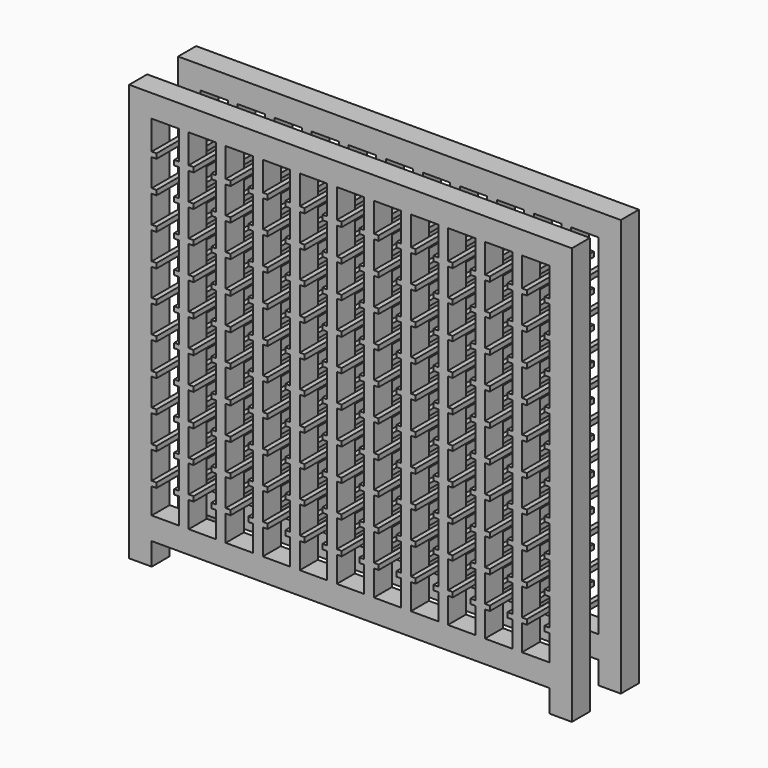
from build123d import *

# Parameters (mm, degrees)
F0_W          = 1568.45
F0_H          = 88.9
F1_DEPTH      = 88.9
F2_W          = 38.1
F2_H          = 1377.95
F3_DEPTH      = 88.9
F6_W          = 19.05
F6_H          = 19.05
F7_DEPTH      = 165.1
F7_DEPTH_BACK = 165.1


with BuildPart() as f1:
    # F0 (on Front) → F1 (new body)
    with BuildSketch(Plane.XZ):
        Polygon((0, 1644.65), (0, 0), (88.9, 0), (88.9, 88.9), (88.9, 177.8), (88.9, 1555.75), (88.9, 1644.65), align=None)
        with Locations((873.125, 133.35)):
            Rectangle(F0_W, F0_H)
        with Locations((873.125, 1600.2)):
            Rectangle(F0_W, F0_H)
        Polygon((1657.35, 177.8), (1657.35, 88.9), (1657.35, 0), (1746.25, 0), (1746.25, 1644.65), (1657.35, 1644.65), (1657.35, 1555.75), align=None)
    extrude(amount=F1_DEPTH)

    # F2 (on face) → F3 (join)
    with BuildSketch(Plane.XZ.offset(88.9)):
        Polygon((1746.25, 1644.65), (0, 1644.65), (0, 0), (88.9, 0), (88.9, 88.9), (1657.35, 88.9), (1657.35, 0), (1746.25, 0), align=None)
        Polygon((88.9, 1555.75), (196.85, 1555.75), (234.95, 1555.75), (342.9, 1555.75), (381, 1555.75), (488.95, 1555.75), (527.05, 1555.75), (635, 1555.75), (673.1, 1555.75), (781.05, 1555.75), (819.15, 1555.75), (927.1, 1555.75), (965.2, 1555.75), (1073.15, 1555.75), (1111.25, 1555.75), (1219.2, 1555.75), (1257.3, 1555.75), (1365.25, 1555.75), (1403.35, 1555.75), (1511.3, 1555.75), (1549.4, 1555.75), (1657.35, 1555.75), (1657.35, 177.8), (1549.4, 177.8), (1511.3, 177.8), (1403.35, 177.8), (1365.25, 177.8), (1257.3, 177.8), (1219.2, 177.8), (1111.25, 177.8), (1073.15, 177.8), (965.2, 177.8), (927.1, 177.8), (819.15, 177.8), (781.05, 177.8), (673.1, 177.8), (635, 177.8), (527.05, 177.8), (488.95, 177.8), (381, 177.8), (342.9, 177.8), (234.95, 177.8), (196.85, 177.8), (88.9, 177.8), align=None, mode=Mode.SUBTRACT)
        with Locations((215.9, 866.775)):
            Rectangle(F2_W, F2_H)
        with Locations((361.95, 866.775)):
            Rectangle(F2_W, F2_H)
        with Locations((508, 866.775)):
            Rectangle(F2_W, F2_H)
        with Locations((654.05, 866.775)):
            Rectangle(F2_W, F2_H)
        with Locations((800.1, 866.775)):
            Rectangle(F2_W, F2_H)
        with Locations((946.15, 866.775)):
            Rectangle(F2_W, F2_H)
        with Locations((1092.2, 866.775)):
            Rectangle(F2_W, F2_H)
        with Locations((1238.25, 866.775)):
            Rectangle(F2_W, F2_H)
        with Locations((1384.3, 866.775)):
            Rectangle(F2_W, F2_H)
        with Locations((1530.35, 866.775)):
            Rectangle(F2_W, F2_H)
    extrude(amount=-F3_DEPTH)


with BuildPart() as f5_1:
    # F5: instance of F1
    add(f1.part.mirror(Plane(origin=(873.125, 76.2, 854.9186148301), x_dir=(1, 0, 0), z_dir=(0, -1, 0))))


with BuildPart() as f1_1:
    add(f1.part)

    add(f5_1.part)  # F7 merges F5_1
    # F6 (on offset) → F7 (join, two sides)
    with BuildSketch(Plane.XZ.offset(-76.2)) as f7_sk:
        with Locations((98.425, 288.925)):
            Rectangle(F6_W, F6_H)
        with Locations((98.425, 415.925)):
            Rectangle(F6_W, F6_H)
        with Locations((98.425, 542.925)):
            Rectangle(F6_W, F6_H)
        with Locations((98.425, 669.925)):
            Rectangle(F6_W, F6_H)
        with Locations((98.425, 796.925)):
            Rectangle(F6_W, F6_H)
        with Locations((98.425, 923.925)):
            Rectangle(F6_W, F6_H)
        with Locations((98.425, 1050.925)):
            Rectangle(F6_W, F6_H)
        with Locations((98.425, 1177.925)):
            Rectangle(F6_W, F6_H)
        with Locations((98.425, 1304.925)):
            Rectangle(F6_W, F6_H)
        with Locations((244.475, 288.925)):
            Rectangle(F6_W, F6_H)
        with Locations((244.475, 415.925)):
            Rectangle(F6_W, F6_H)
        with Locations((244.475, 542.925)):
            Rectangle(F6_W, F6_H)
        with Locations((244.475, 669.925)):
            Rectangle(F6_W, F6_H)
        with Locations((244.475, 796.925)):
            Rectangle(F6_W, F6_H)
        with Locations((244.475, 923.925)):
            Rectangle(F6_W, F6_H)
        with Locations((244.475, 1050.925)):
            Rectangle(F6_W, F6_H)
        with Locations((244.475, 1177.925)):
            Rectangle(F6_W, F6_H)
        with Locations((244.475, 1304.925)):
            Rectangle(F6_W, F6_H)
        with Locations((390.525, 288.925)):
            Rectangle(F6_W, F6_H)
        with Locations((390.525, 415.925)):
            Rectangle(F6_W, F6_H)
        with Locations((390.525, 542.925)):
            Rectangle(F6_W, F6_H)
        with Locations((390.525, 669.925)):
            Rectangle(F6_W, F6_H)
        with Locations((390.525, 796.925)):
            Rectangle(F6_W, F6_H)
        with Locations((390.525, 923.925)):
            Rectangle(F6_W, F6_H)
        with Locations((390.525, 1050.925)):
            Rectangle(F6_W, F6_H)
        with Locations((390.525, 1177.925)):
            Rectangle(F6_W, F6_H)
        with Locations((390.525, 1304.925)):
            Rectangle(F6_W, F6_H)
        with Locations((536.575, 288.925)):
            Rectangle(F6_W, F6_H)
        with Locations((536.575, 415.925)):
            Rectangle(F6_W, F6_H)
        with Locations((536.575, 542.925)):
            Rectangle(F6_W, F6_H)
        with Locations((536.575, 669.925)):
            Rectangle(F6_W, F6_H)
        with Locations((536.575, 796.925)):
            Rectangle(F6_W, F6_H)
        with Locations((536.575, 923.925)):
            Rectangle(F6_W, F6_H)
        with Locations((536.575, 1050.925)):
            Rectangle(F6_W, F6_H)
        with Locations((536.575, 1177.925)):
            Rectangle(F6_W, F6_H)
        with Locations((536.575, 1304.925)):
            Rectangle(F6_W, F6_H)
        with Locations((682.625, 288.925)):
            Rectangle(F6_W, F6_H)
        with Locations((682.625, 415.925)):
            Rectangle(F6_W, F6_H)
        with Locations((682.625, 542.925)):
            Rectangle(F6_W, F6_H)
        with Locations((682.625, 669.925)):
            Rectangle(F6_W, F6_H)
        with Locations((682.625, 796.925)):
            Rectangle(F6_W, F6_H)
        with Locations((682.625, 923.925)):
            Rectangle(F6_W, F6_H)
        with Locations((682.625, 1050.925)):
            Rectangle(F6_W, F6_H)
        with Locations((682.625, 1177.925)):
            Rectangle(F6_W, F6_H)
        with Locations((682.625, 1304.925)):
            Rectangle(F6_W, F6_H)
        with Locations((828.675, 288.925)):
            Rectangle(F6_W, F6_H)
        with Locations((828.675, 415.925)):
            Rectangle(F6_W, F6_H)
        with Locations((828.675, 542.925)):
            Rectangle(F6_W, F6_H)
        with Locations((828.675, 669.925)):
            Rectangle(F6_W, F6_H)
        with Locations((828.675, 796.925)):
            Rectangle(F6_W, F6_H)
        with Locations((828.675, 923.925)):
            Rectangle(F6_W, F6_H)
        with Locations((828.675, 1050.925)):
            Rectangle(F6_W, F6_H)
        with Locations((828.675, 1177.925)):
            Rectangle(F6_W, F6_H)
        with Locations((828.675, 1304.925)):
            Rectangle(F6_W, F6_H)
        with Locations((974.725, 288.925)):
            Rectangle(F6_W, F6_H)
        with Locations((974.725, 415.925)):
            Rectangle(F6_W, F6_H)
        with Locations((974.725, 542.925)):
            Rectangle(F6_W, F6_H)
        with Locations((974.725, 669.925)):
            Rectangle(F6_W, F6_H)
        with Locations((974.725, 796.925)):
            Rectangle(F6_W, F6_H)
        with Locations((974.725, 923.925)):
            Rectangle(F6_W, F6_H)
        with Locations((974.725, 1050.925)):
            Rectangle(F6_W, F6_H)
        with Locations((974.725, 1177.925)):
            Rectangle(F6_W, F6_H)
        with Locations((974.725, 1304.925)):
            Rectangle(F6_W, F6_H)
        with Locations((1120.775, 288.925)):
            Rectangle(F6_W, F6_H)
        with Locations((1120.775, 415.925)):
            Rectangle(F6_W, F6_H)
        with Locations((1120.775, 542.925)):
            Rectangle(F6_W, F6_H)
        with Locations((1120.775, 669.925)):
            Rectangle(F6_W, F6_H)
        with Locations((1120.775, 796.925)):
            Rectangle(F6_W, F6_H)
        with Locations((1120.775, 923.925)):
            Rectangle(F6_W, F6_H)
        with Locations((1120.775, 1050.925)):
            Rectangle(F6_W, F6_H)
        with Locations((1120.775, 1177.925)):
            Rectangle(F6_W, F6_H)
        with Locations((1120.775, 1304.925)):
            Rectangle(F6_W, F6_H)
        with Locations((1266.825, 288.925)):
            Rectangle(F6_W, F6_H)
        with Locations((1266.825, 415.925)):
            Rectangle(F6_W, F6_H)
        with Locations((1266.825, 542.925)):
            Rectangle(F6_W, F6_H)
        with Locations((1266.825, 669.925)):
            Rectangle(F6_W, F6_H)
        with Locations((1266.825, 796.925)):
            Rectangle(F6_W, F6_H)
        with Locations((1266.825, 923.925)):
            Rectangle(F6_W, F6_H)
        with Locations((1266.825, 1050.925)):
            Rectangle(F6_W, F6_H)
        with Locations((1266.825, 1177.925)):
            Rectangle(F6_W, F6_H)
        with Locations((1266.825, 1304.925)):
            Rectangle(F6_W, F6_H)
        with Locations((1412.875, 288.925)):
            Rectangle(F6_W, F6_H)
        with Locations((1412.875, 415.925)):
            Rectangle(F6_W, F6_H)
        with Locations((1412.875, 542.925)):
            Rectangle(F6_W, F6_H)
        with Locations((1412.875, 669.925)):
            Rectangle(F6_W, F6_H)
        with Locations((1412.875, 796.925)):
            Rectangle(F6_W, F6_H)
        with Locations((1412.875, 923.925)):
            Rectangle(F6_W, F6_H)
        with Locations((1412.875, 1050.925)):
            Rectangle(F6_W, F6_H)
        with Locations((1412.875, 1177.925)):
            Rectangle(F6_W, F6_H)
        with Locations((1412.875, 1304.925)):
            Rectangle(F6_W, F6_H)
        with Locations((1558.925, 288.925)):
            Rectangle(F6_W, F6_H)
        with Locations((1558.925, 415.925)):
            Rectangle(F6_W, F6_H)
        with Locations((1558.925, 542.925)):
            Rectangle(F6_W, F6_H)
        with Locations((1558.925, 669.925)):
            Rectangle(F6_W, F6_H)
        with Locations((1558.925, 796.925)):
            Rectangle(F6_W, F6_H)
        with Locations((1558.925, 923.925)):
            Rectangle(F6_W, F6_H)
        with Locations((1558.925, 1050.925)):
            Rectangle(F6_W, F6_H)
        with Locations((1558.925, 1177.925)):
            Rectangle(F6_W, F6_H)
        with Locations((1558.925, 1304.925)):
            Rectangle(F6_W, F6_H)
        with Locations((98.425, 1431.925)):
            Rectangle(F6_W, F6_H)
        with Locations((244.475, 1431.925)):
            Rectangle(F6_W, F6_H)
        with Locations((390.525, 1431.925)):
            Rectangle(F6_W, F6_H)
        with Locations((536.575, 1431.925)):
            Rectangle(F6_W, F6_H)
        with Locations((682.625, 1431.925)):
            Rectangle(F6_W, F6_H)
        with Locations((828.675, 1431.925)):
            Rectangle(F6_W, F6_H)
        with Locations((974.725, 1431.925)):
            Rectangle(F6_W, F6_H)
        with Locations((1120.775, 1431.925)):
            Rectangle(F6_W, F6_H)
        with Locations((1266.825, 1431.925)):
            Rectangle(F6_W, F6_H)
        with Locations((1412.875, 1431.925)):
            Rectangle(F6_W, F6_H)
        with Locations((1558.925, 1431.925)):
            Rectangle(F6_W, F6_H)
        with Locations((187.325, 288.925)):
            Rectangle(F6_W, F6_H)
        with Locations((187.325, 415.925)):
            Rectangle(F6_W, F6_H)
        with Locations((187.325, 542.925)):
            Rectangle(F6_W, F6_H)
        with Locations((187.325, 669.925)):
            Rectangle(F6_W, F6_H)
        with Locations((187.325, 796.925)):
            Rectangle(F6_W, F6_H)
        with Locations((187.325, 923.925)):
            Rectangle(F6_W, F6_H)
        with Locations((187.325, 1050.925)):
            Rectangle(F6_W, F6_H)
        with Locations((187.325, 1177.925)):
            Rectangle(F6_W, F6_H)
        with Locations((187.325, 1304.925)):
            Rectangle(F6_W, F6_H)
        with Locations((187.325, 1431.925)):
            Rectangle(F6_W, F6_H)
        with Locations((333.375, 288.925)):
            Rectangle(F6_W, F6_H)
        with Locations((333.375, 415.925)):
            Rectangle(F6_W, F6_H)
        with Locations((333.375, 542.925)):
            Rectangle(F6_W, F6_H)
        with Locations((333.375, 669.925)):
            Rectangle(F6_W, F6_H)
        with Locations((333.375, 796.925)):
            Rectangle(F6_W, F6_H)
        with Locations((333.375, 923.925)):
            Rectangle(F6_W, F6_H)
        with Locations((333.375, 1050.925)):
            Rectangle(F6_W, F6_H)
        with Locations((333.375, 1177.925)):
            Rectangle(F6_W, F6_H)
        with Locations((333.375, 1304.925)):
            Rectangle(F6_W, F6_H)
        with Locations((333.375, 1431.925)):
            Rectangle(F6_W, F6_H)
        with Locations((479.425, 288.925)):
            Rectangle(F6_W, F6_H)
        with Locations((479.425, 415.925)):
            Rectangle(F6_W, F6_H)
        with Locations((479.425, 542.925)):
            Rectangle(F6_W, F6_H)
        with Locations((479.425, 669.925)):
            Rectangle(F6_W, F6_H)
        with Locations((479.425, 796.925)):
            Rectangle(F6_W, F6_H)
        with Locations((479.425, 923.925)):
            Rectangle(F6_W, F6_H)
        with Locations((479.425, 1050.925)):
            Rectangle(F6_W, F6_H)
        with Locations((479.425, 1177.925)):
            Rectangle(F6_W, F6_H)
        with Locations((479.425, 1304.925)):
            Rectangle(F6_W, F6_H)
        with Locations((479.425, 1431.925)):
            Rectangle(F6_W, F6_H)
        with Locations((625.475, 288.925)):
            Rectangle(F6_W, F6_H)
        with Locations((625.475, 415.925)):
            Rectangle(F6_W, F6_H)
        with Locations((625.475, 542.925)):
            Rectangle(F6_W, F6_H)
        with Locations((625.475, 669.925)):
            Rectangle(F6_W, F6_H)
        with Locations((625.475, 796.925)):
            Rectangle(F6_W, F6_H)
        with Locations((625.475, 923.925)):
            Rectangle(F6_W, F6_H)
        with Locations((625.475, 1050.925)):
            Rectangle(F6_W, F6_H)
        with Locations((625.475, 1177.925)):
            Rectangle(F6_W, F6_H)
        with Locations((625.475, 1304.925)):
            Rectangle(F6_W, F6_H)
        with Locations((625.475, 1431.925)):
            Rectangle(F6_W, F6_H)
        with Locations((771.525, 288.925)):
            Rectangle(F6_W, F6_H)
        with Locations((771.525, 415.925)):
            Rectangle(F6_W, F6_H)
        with Locations((771.525, 542.925)):
            Rectangle(F6_W, F6_H)
        with Locations((771.525, 669.925)):
            Rectangle(F6_W, F6_H)
        with Locations((771.525, 796.925)):
            Rectangle(F6_W, F6_H)
        with Locations((771.525, 923.925)):
            Rectangle(F6_W, F6_H)
        with Locations((771.525, 1050.925)):
            Rectangle(F6_W, F6_H)
        with Locations((771.525, 1177.925)):
            Rectangle(F6_W, F6_H)
        with Locations((771.525, 1304.925)):
            Rectangle(F6_W, F6_H)
        with Locations((771.525, 1431.925)):
            Rectangle(F6_W, F6_H)
        with Locations((917.575, 288.925)):
            Rectangle(F6_W, F6_H)
        with Locations((917.575, 415.925)):
            Rectangle(F6_W, F6_H)
        with Locations((917.575, 542.925)):
            Rectangle(F6_W, F6_H)
        with Locations((917.575, 669.925)):
            Rectangle(F6_W, F6_H)
        with Locations((917.575, 796.925)):
            Rectangle(F6_W, F6_H)
        with Locations((917.575, 923.925)):
            Rectangle(F6_W, F6_H)
        with Locations((917.575, 1050.925)):
            Rectangle(F6_W, F6_H)
        with Locations((917.575, 1177.925)):
            Rectangle(F6_W, F6_H)
        with Locations((917.575, 1304.925)):
            Rectangle(F6_W, F6_H)
        with Locations((917.575, 1431.925)):
            Rectangle(F6_W, F6_H)
        with Locations((1063.625, 288.925)):
            Rectangle(F6_W, F6_H)
        with Locations((1063.625, 415.925)):
            Rectangle(F6_W, F6_H)
        with Locations((1063.625, 542.925)):
            Rectangle(F6_W, F6_H)
        with Locations((1063.625, 669.925)):
            Rectangle(F6_W, F6_H)
        with Locations((1063.625, 796.925)):
            Rectangle(F6_W, F6_H)
        with Locations((1063.625, 923.925)):
            Rectangle(F6_W, F6_H)
        with Locations((1063.625, 1050.925)):
            Rectangle(F6_W, F6_H)
        with Locations((1063.625, 1177.925)):
            Rectangle(F6_W, F6_H)
        with Locations((1063.625, 1304.925)):
            Rectangle(F6_W, F6_H)
        with Locations((1063.625, 1431.925)):
            Rectangle(F6_W, F6_H)
        with Locations((1209.675, 288.925)):
            Rectangle(F6_W, F6_H)
        with Locations((1209.675, 415.925)):
            Rectangle(F6_W, F6_H)
        with Locations((1209.675, 542.925)):
            Rectangle(F6_W, F6_H)
        with Locations((1209.675, 669.925)):
            Rectangle(F6_W, F6_H)
        with Locations((1209.675, 796.925)):
            Rectangle(F6_W, F6_H)
        with Locations((1209.675, 923.925)):
            Rectangle(F6_W, F6_H)
        with Locations((1209.675, 1050.925)):
            Rectangle(F6_W, F6_H)
        with Locations((1209.675, 1177.925)):
            Rectangle(F6_W, F6_H)
        with Locations((1209.675, 1304.925)):
            Rectangle(F6_W, F6_H)
        with Locations((1209.675, 1431.925)):
            Rectangle(F6_W, F6_H)
        with Locations((1355.725, 288.925)):
            Rectangle(F6_W, F6_H)
        with Locations((1355.725, 415.925)):
            Rectangle(F6_W, F6_H)
        with Locations((1355.725, 542.925)):
            Rectangle(F6_W, F6_H)
        with Locations((1355.725, 669.925)):
            Rectangle(F6_W, F6_H)
        with Locations((1355.725, 796.925)):
            Rectangle(F6_W, F6_H)
        with Locations((1355.725, 923.925)):
            Rectangle(F6_W, F6_H)
        with Locations((1355.725, 1050.925)):
            Rectangle(F6_W, F6_H)
        with Locations((1355.725, 1177.925)):
            Rectangle(F6_W, F6_H)
        with Locations((1355.725, 1304.925)):
            Rectangle(F6_W, F6_H)
        with Locations((1355.725, 1431.925)):
            Rectangle(F6_W, F6_H)
        with Locations((1501.775, 288.925)):
            Rectangle(F6_W, F6_H)
        with Locations((1501.775, 415.925)):
            Rectangle(F6_W, F6_H)
        with Locations((1501.775, 542.925)):
            Rectangle(F6_W, F6_H)
        with Locations((1501.775, 669.925)):
            Rectangle(F6_W, F6_H)
        with Locations((1501.775, 796.925)):
            Rectangle(F6_W, F6_H)
        with Locations((1501.775, 923.925)):
            Rectangle(F6_W, F6_H)
        with Locations((1501.775, 1050.925)):
            Rectangle(F6_W, F6_H)
        with Locations((1501.775, 1177.925)):
            Rectangle(F6_W, F6_H)
        with Locations((1501.775, 1304.925)):
            Rectangle(F6_W, F6_H)
        with Locations((1501.775, 1431.925)):
            Rectangle(F6_W, F6_H)
        with Locations((1647.825, 288.925)):
            Rectangle(F6_W, F6_H)
        with Locations((1647.825, 415.925)):
            Rectangle(F6_W, F6_H)
        with Locations((1647.825, 542.925)):
            Rectangle(F6_W, F6_H)
        with Locations((1647.825, 669.925)):
            Rectangle(F6_W, F6_H)
        with Locations((1647.825, 796.925)):
            Rectangle(F6_W, F6_H)
        with Locations((1647.825, 923.925)):
            Rectangle(F6_W, F6_H)
        with Locations((1647.825, 1050.925)):
            Rectangle(F6_W, F6_H)
        with Locations((1647.825, 1177.925)):
            Rectangle(F6_W, F6_H)
        with Locations((1647.825, 1304.925)):
            Rectangle(F6_W, F6_H)
        with Locations((1647.825, 1431.925)):
            Rectangle(F6_W, F6_H)
    extrude(amount=F7_DEPTH)
    extrude(f7_sk.sketch, amount=-F7_DEPTH_BACK)


solid = f1_1.part
